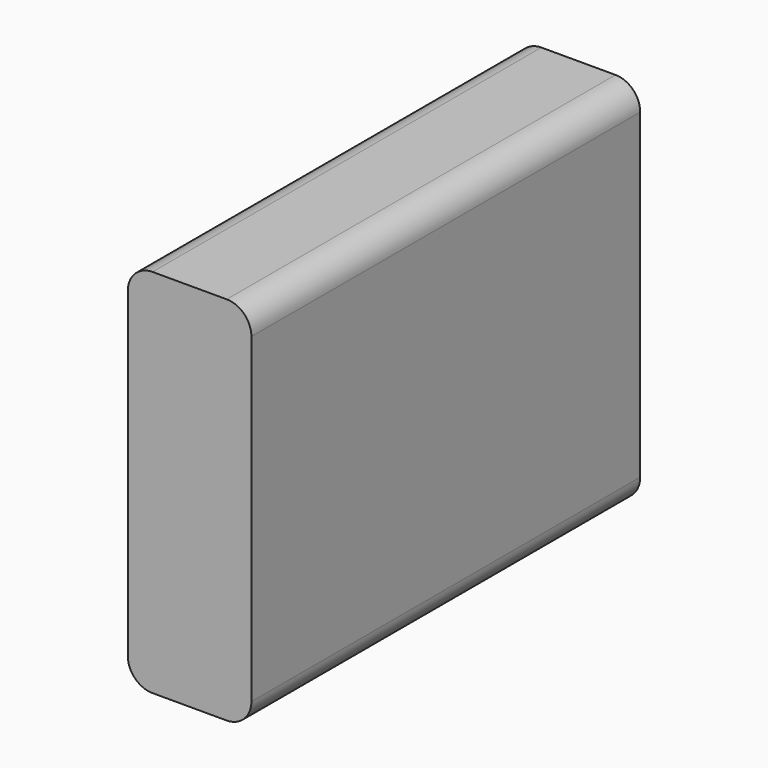
from build123d import *

# Parameters (mm, degrees)
F0_W          = 99.8685956001
F0_H          = 76.2
F1_DEPTH      = 25.4
F2_R          = 5.08
F3_R          = 5.08
F4_R          = 5.08
F5_R          = 5.08
F6_W          = 7
F6_H          = 13.8
F7_DEPTH      = 15
F8_W          = 14.7339338437
F8_H          = 1.7859311774
F9_DEPTH      = 15
F11_DEPTH     = 5
F12_T4_DEPTH  = 32.018367851
F12_T10_DEPTH = 32.018367851
F12_T17_DEPTH = 32.018367851
F12_T23_DEPTH = 32.018367851


# Not quite as in the source:
# - a fillet or chamfer that OpenCascade refuses, or shapes differently, is made with other operations: its cross-section is extruded or revolved along the edge and cut away or added


with BuildPart() as f1:
    # F0 (on Right) → F1 (new body)
    with BuildSketch(Plane.YZ):
        Rectangle(F0_W, F0_H)
    extrude(amount=F1_DEPTH)

    # F2
    f2_edges = [f1.edges().sort_by_distance(p)[0] for p in [
        (25.4, 0, 38.1),
    ]]
    fillet(f2_edges, radius=F2_R)

    # F3
    f3_edges = [f1.edges().sort_by_distance(p)[0] for p in [
        (0, 0, 38.1),
    ]]
    fillet(f3_edges, radius=F3_R)

    # F4
    f4_edges = [f1.edges().sort_by_distance(p)[0] for p in [
        (25.4, 0, -38.1),
    ]]
    fillet(f4_edges, radius=F4_R)

    # F5
    f5_edges = [f1.edges().sort_by_distance(p)[0] for p in [
        (0, 0, -38.1),
    ]]
    fillet(f5_edges, radius=F5_R)

    # F6 (on face) → F7 (cut)
    with BuildSketch(Plane(origin=(0, 49.9342978001, 0), x_dir=(-1, 0, 0), z_dir=(0, 1, 0))):
        with Locations((-6.8276954116, 20.0042553112)):
            Rectangle(F6_W, F6_H)
        with Locations((-16.8951429576, 20.0042553112)):
            Rectangle(F6_W, F6_H)
    extrude(amount=-F7_DEPTH, mode=Mode.SUBTRACT)

    # F8 (on face) → F9 (cut)
    with BuildSketch(Plane(origin=(0, 49.9342978001, 0), x_dir=(-1, 0, 0), z_dir=(0, 1, 0))):
        with Locations((-11.9025348686, 11.1820721067)):
            Rectangle(F8_W, F8_H)
        Polygon((-4.5355679467, 10.289106518), (-19.2695017904, 10.289106518), (-17.8024861962, 8.3756083623), (-5.9387991205, 8.3756083623), align=None)
    extrude(amount=-F9_DEPTH, mode=Mode.SUBTRACT)

    # F10 (on face) → F11 (cut)
    with BuildSketch(Plane(origin=(0, 49.9342978001, 0), x_dir=(-1, 0, 0), z_dir=(0, 1, 0))):
        Polygon((-16.0813947992, -32.9593643546), (-9.4630269482, -32.9593643546), (-4.3930630334, -28.7051595036), (-3.2437955169, -22.1873395316), (-6.5529794424, -16.4556648411), (-12.7722108737, -14.1920497201), (-18.9914423049, -16.4556648411), (-22.3006262304, -22.1873395316), (-21.151358714, -28.7051595036), align=None)
    extrude(amount=-F11_DEPTH, mode=Mode.SUBTRACT)

    # F12: fillet of radius 5.08 on 4 edges, made by hand


with BuildPart() as f12_tool2:
    # F12_s3 → F12_t4 (new body)
    with BuildSketch(Plane(origin=(5.5233724705, 0, -9.566761748), x_dir=(0, 1, 0), z_dir=(0.5, 0, -0.8660254038))):
        with BuildLine():
            ThreePointArc((50.0142978001, 8.21923907), (46.4221953516, 6.7313415185), (44.9342978001, 3.13923907))
            Line((44.9342978001, 3.13923907), (44.9342978001, 8.21923907))
            Line((44.9342978001, 8.21923907), (50.0142978001, 8.21923907))
        make_face()
    extrude(amount=F12_T4_DEPTH)

    split(bisect_by=Plane.XZ.offset(-49.9342978001), keep=Keep.TOP)

    split(bisect_by=Plane(origin=(25.4224385924, 0, -4.4826618392), x_dir=(0, 1, 0), z_dir=(-0.984807753, 0, 0.1736481777)), keep=Keep.TOP)


with BuildPart() as f1_1:
    add(f1.part)

    # F12_t1: union F12_tool2
    add(f12_tool2.part)


with BuildPart() as f12_tool8:
    # F12_s9 → F12_t10 (new body)
    with BuildSketch(Plane(origin=(31.5112153695, 0, -26.4410491945), x_dir=(0, 1, 0), z_dir=(-0.7660444431, 0, 0.6427876097))):
        with BuildLine():
            ThreePointArc((50.0142978001, 19.1656214402), (46.4221953516, 17.6777238886), (44.9342978001, 14.0856214402))
            Line((44.9342978001, 14.0856214402), (44.9342978001, 19.1656214402))
            Line((44.9342978001, 19.1656214402), (50.0142978001, 19.1656214402))
        make_face()
    extrude(amount=F12_T10_DEPTH)

    split(bisect_by=Plane.XZ.offset(-49.9342978001), keep=Keep.TOP)

    split(bisect_by=Plane(origin=(-0.6482754096, 0, -0.1143084456), x_dir=(0, 1, 0), z_dir=(0.984807753, 0, 0.1736481777)), keep=Keep.TOP)

    split(bisect_by=Plane.XY.offset(-32.9593643546), keep=Keep.TOP)


with BuildPart() as f1_2:
    add(f1_1.part)

    # F12_t7: union F12_tool8
    add(f12_tool8.part)


with BuildPart() as f12_tool15:
    # F12_s16 → F12_t17 (new body)
    with BuildSketch(Plane(origin=(-15.1464509592, 0, -26.2344226156), x_dir=(0, 1, 0), z_dir=(0.5, 0, 0.8660254038))):
        with BuildLine():
            ThreePointArc((50.0142978001, -13.9028790881), (46.4221953516, -15.3907766397), (44.9342978001, -18.9828790881))
            Line((44.9342978001, -18.9828790881), (44.9342978001, -13.9028790881))
            Line((44.9342978001, -13.9028790881), (50.0142978001, -13.9028790881))
        make_face()
    extrude(amount=F12_T17_DEPTH)

    split(bisect_by=Plane.XZ.offset(-49.9342978001), keep=Keep.TOP)

    split(bisect_by=Plane(origin=(-12.3194239937, 0, -14.6817178032), x_dir=(0, 1, 0), z_dir=(0.6427876097, 0, 0.7660444431)), keep=Keep.TOP)


with BuildPart() as f1_3:
    add(f1_2.part)

    # F12_t14: union F12_tool15
    add(f12_tool15.part)


with BuildPart() as f12_tool21:
    # F12_s22 → F12_t23 (new body)
    with BuildSketch(Plane(origin=(8.0063594172, 0, 6.7181332341), x_dir=(0, 1, 0), z_dir=(-0.7660444431, 0, -0.6427876097))):
        with BuildLine():
            ThreePointArc((50.0142978001, 35.585259236), (46.4221953516, 34.0973616844), (44.9342978001, 30.505259236))
            Line((44.9342978001, 30.505259236), (44.9342978001, 35.585259236))
            Line((44.9342978001, 35.585259236), (50.0142978001, 35.585259236))
        make_face()
    extrude(amount=F12_T23_DEPTH)

    split(bisect_by=Plane.XZ.offset(-49.9342978001), keep=Keep.TOP)

    split(bisect_by=Plane(origin=(7.1180698344, 0, 4.109619535), x_dir=(0, 1, 0), z_dir=(-0.8660254038, 0, -0.5)), keep=Keep.TOP)

    split(bisect_by=Plane.XY.offset(-32.9593643546), keep=Keep.TOP)


with BuildPart() as f1_4:
    add(f1_3.part)

    # F12_t20: union F12_tool21
    add(f12_tool21.part)


solid = f1_4.part
